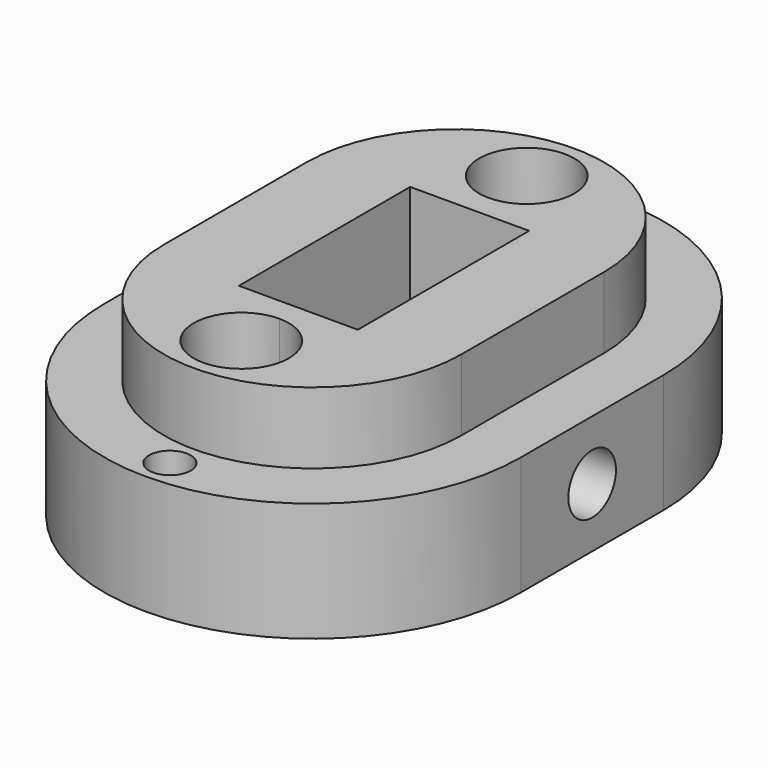
from build123d import *

# Parameters (mm, degrees)
F0_W      = 25
F0_H      = 15
F1_DEPTH  = 6
F3_DEPTH  = 10
F5_D      = 5
F6_W      = 10
F6_H      = 15
F7_DEPTH  = 16
F8_DEPTH  = 25.4
F9_DEPTH  = 10
F10_R     = 1.75
F11_DEPTH = 10


with BuildPart() as f1:
    # F0 (on Top) → F1 (new body)
    with BuildSketch(Plane.XY):
        with BuildLine():
            ThreePointArc((-22.1608236432, 15), (-34.6608236432, 27.5), (-47.1608236432, 15))
            Line((-47.1608236432, 15), (-22.1608236432, 15))
        make_face()
        with Locations((-34.6608236432, 7.5)):
            Rectangle(F0_W, F0_H)
        with BuildLine():
            Line((-22.1608236432, 0), (-47.1608236432, 0))
            ThreePointArc((-47.1608236432, 0), (-34.6608236432, -12.5), (-22.1608236432, 0))
        make_face()
    extrude(amount=F1_DEPTH)

    # F2 (on Top) → F3 (join)
    with BuildSketch(Plane.XY):
        with BuildLine():
            Line((-17.1608236432, 0), (-17.1608236432, 15))
            ThreePointArc((-17.1608236432, 15), (-34.6608236432, 32.5), (-52.1608236432, 15))
            Line((-52.1608236432, 15), (-52.1608236432, 0))
            ThreePointArc((-52.1608236432, 0), (-34.6608236432, -17.5), (-17.1608236432, 0))
        make_face()
    extrude(amount=-F3_DEPTH)

    # F5 (through all)
    with Locations(Plane(origin=(-52.1608236432, 0, 0), x_dir=(0, -1, 0), z_dir=(-1, 0, 0))):
        with Locations((-7.5, -5)):
            Hole(F5_D / 2)

    # F6 (on face) → F7 (cut, through all)
    with BuildSketch(Plane(origin=(0, 0, -10), x_dir=(1, 0, 0), z_dir=(0, 0, -1))):
        Polygon((-39.6608236432, 1.5), (-39.6608236432, 0), (-29.6608236432, 0), (-29.6608236432, 1.5), (-34.6608236432, 1.5), align=None)
        with Locations((-34.6608236432, -7.5)):
            Rectangle(F6_W, F6_H)
        Polygon((-29.6608236432, -15), (-39.6608236432, -15), (-39.6608236432, -16.5), (-34.6608236432, -16.5), (-29.6608236432, -16.5), align=None)
    extrude(amount=-F7_DEPTH, mode=Mode.SUBTRACT)

    # F6 (on face) → F8 (cut)
    with BuildSketch(Plane(origin=(0, 0, -10), x_dir=(1, 0, 0), z_dir=(0, 0, -1))):
        with BuildLine():
            ThreePointArc((-30.6608236432, -22.5), (-31.8323965185, -19.6715728753), (-34.6608236432, -18.5))
            ThreePointArc((-34.6608236432, -18.5), (-37.489250768, -25.3284271247), (-30.6608236432, -22.5))
        make_face()
        with BuildLine():
            ThreePointArc((-30.6608236432, 7.5), (-37.489250768, 10.3284271247), (-34.6608236432, 3.5))
            ThreePointArc((-34.6608236432, 3.5), (-31.8323965185, 4.6715728753), (-30.6608236432, 7.5))
        make_face()
    extrude(amount=-F8_DEPTH, mode=Mode.SUBTRACT)

    # F6 (on face) → F9 (join)
    with BuildSketch(Plane(origin=(0, 0, -10), x_dir=(1, 0, 0), z_dir=(0, 0, -1))):
        with BuildLine():
            ThreePointArc((-30.6608236432, -22.5), (-31.8323965185, -19.6715728753), (-34.6608236432, -18.5))
            ThreePointArc((-34.6608236432, -18.5), (-37.489250768, -25.3284271247), (-30.6608236432, -22.5))
        make_face()
        with BuildLine():
            ThreePointArc((-30.6608236432, 7.5), (-37.489250768, 10.3284271247), (-34.6608236432, 3.5))
            ThreePointArc((-34.6608236432, 3.5), (-31.8323965185, 4.6715728753), (-30.6608236432, 7.5))
        make_face()
    extrude(amount=-F9_DEPTH)

    # F10 (on face) → F11 (cut)
    with BuildSketch(Plane.XY):
        with Locations((-34.6608236432, 30)):
            Circle(F10_R)
        with Locations((-34.6608236432, -15)):
            Circle(F10_R)
    extrude(amount=-F11_DEPTH, mode=Mode.SUBTRACT)


solid = f1.part
